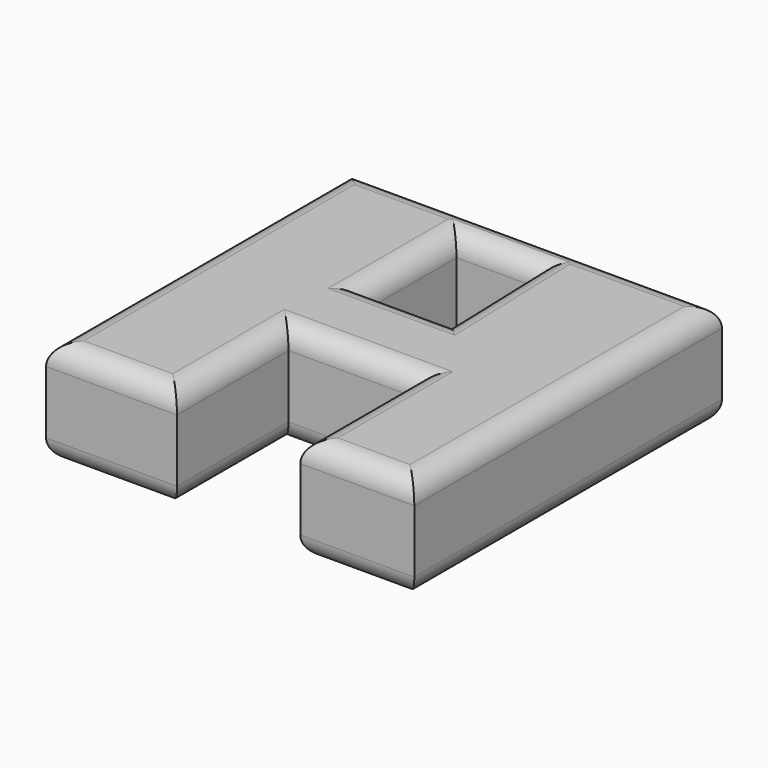
from build123d import *

# Parameters (mm, degrees)
F1_DEPTH      = 15
F2_T1_DEPTH   = 68.2414875925
F2_T3_DEPTH   = 69.4962510467
F2_T5_DEPTH   = 33.7555244192
F2_T7_DEPTH   = 27.4655555189
F2_T9_DEPTH   = 18.1505084038
F2_T11_DEPTH  = 28.0705761909
F2_T13_DEPTH  = 31.3354547694
F2_T15_DEPTH  = 70.1012717187
F2_T17_DEPTH  = 16.2727097049
F2_T22_DEPTH  = 19.0483759437
F2_T27_DEPTH  = 31.281174035
F2_T33_DEPTH  = 19.5733014774
F2_T38_DEPTH  = 19.0483759437
F2_T43_DEPTH  = 31.281174035
F2_T49_DEPTH  = 19.5733014774
F2_T55_DEPTH  = 25.6505084038
F2_T59_DEPTH  = 34.9655555189
F2_T66_DEPTH  = 35.5705761909
F2_T70_DEPTH  = 25.6505084038
F2_T77_DEPTH  = 23.7727097049
F2_T81_DEPTH  = 26.5483759437
F2_T88_DEPTH  = 31.281174035
F2_T92_DEPTH  = 19.0483759437
F2_T99_DEPTH  = 19.5733014774
F2_T103_DEPTH = 31.281174035
F2_T110_DEPTH = 23.7727097049
F2_T114_DEPTH = 27.0733014774
F2_T121_DEPTH = 34.9655555189
F2_T125_DEPTH = 25.6505084038
F2_T132_DEPTH = 25.6505084038
F2_T136_DEPTH = 35.5705761909
F2_T143_DEPTH = 26.5483759437
F2_T147_DEPTH = 23.7727097049
F2_T154_DEPTH = 19.0483759437
F2_T158_DEPTH = 31.281174035
F2_T165_DEPTH = 31.281174035
F2_T169_DEPTH = 19.5733014774
F2_T176_DEPTH = 27.0733014774
F2_T180_DEPTH = 23.7727097049


# Not quite as in the source:
# - a fillet or chamfer that OpenCascade refuses, or shapes differently, is made with other operations: its cross-section is extruded or revolved along the edge and cut away or added


with BuildPart() as f1:
    # F0 (on Top) → F1 (new body)
    with BuildSketch(Plane.XY):
        Polygon((24.4360174984, 0), (0, 0), (-25.7803853601, 0), (-28.8054700941, 0), (-28.8054700941, -54.4962510467), (-10.0499456748, -54.4962510467), (-10.0499456748, -34.5306955278), (8.1005627289, -34.5306955278), (8.1005627289, -55.1012717187), (24.4360174984, -55.1012717187), align=None)
        Polygon((-9.4178915024, -5.2225748077), (2.1304844413, -5.2225748077), (2.655409975, -21.4952845126), (-9.4178915024, -21.4952845126), align=None, mode=Mode.SUBTRACT)
    extrude(amount=F1_DEPTH)

    # F2: fillet of radius 3 on 24 edges, made by hand

    # F2_s2 → F2_t1 (cut)
    with BuildSketch(Plane.YZ.offset(-36.3054700941)):
        with BuildLine():
            ThreePointArc((0, 12), (-0.8786796564, 14.1213203436), (-3, 15))
            Line((-3, 15), (0, 15))
            Line((0, 15), (0, 12))
        make_face()
        with BuildLine():
            ThreePointArc((0, 3), (-0.8786796564, 0.8786796564), (-3, 0))
            Line((-3, 0), (0, 0))
            Line((0, 0), (0, 3))
        make_face()
    extrude(amount=F2_T1_DEPTH, mode=Mode.SUBTRACT)

    # F2_s4 → F2_t3 (cut)
    with BuildSketch(Plane.XZ.offset(-7.5)):
        with BuildLine():
            ThreePointArc((-28.8054700941, 12), (-27.9267904376, 14.1213203436), (-25.8054700941, 15))
            Line((-25.8054700941, 15), (-28.8054700941, 15))
            Line((-28.8054700941, 15), (-28.8054700941, 12))
        make_face()
        with BuildLine():
            ThreePointArc((-25.8054700941, 0), (-27.9267904376, 0.8786796564), (-28.8054700941, 3))
            Line((-28.8054700941, 3), (-28.8054700941, 0))
            Line((-28.8054700941, 0), (-25.8054700941, 0))
        make_face()
    extrude(amount=F2_T3_DEPTH, mode=Mode.SUBTRACT)

    # F2_s6 → F2_t5 (cut)
    with BuildSketch(Plane.YZ.offset(-36.3054700941)):
        with BuildLine():
            ThreePointArc((-54.4962510467, 12), (-53.6175713902, 14.1213203436), (-51.4962510467, 15))
            Line((-51.4962510467, 15), (-54.4962510467, 15))
            Line((-54.4962510467, 15), (-54.4962510467, 12))
        make_face()
        with BuildLine():
            ThreePointArc((-51.4962510467, 0), (-53.6175713902, 0.8786796564), (-54.4962510467, 3))
            Line((-54.4962510467, 3), (-54.4962510467, 0))
            Line((-54.4962510467, 0), (-51.4962510467, 0))
        make_face()
    extrude(amount=F2_T5_DEPTH, mode=Mode.SUBTRACT)

    # F2_s8 → F2_t7 (cut)
    with BuildSketch(Plane.XZ.offset(34.5306955278)):
        with BuildLine():
            ThreePointArc((-10.0499456748, 12), (-10.9286253313, 14.1213203436), (-13.0499456748, 15))
            Line((-13.0499456748, 15), (-10.0499456748, 15))
            Line((-10.0499456748, 15), (-10.0499456748, 12))
        make_face()
        with BuildLine():
            ThreePointArc((-13.0499456748, 0), (-10.9286253313, 0.8786796564), (-10.0499456748, 3))
            Line((-10.0499456748, 3), (-10.0499456748, 0))
            Line((-10.0499456748, 0), (-13.0499456748, 0))
        make_face()
    extrude(amount=F2_T7_DEPTH, mode=Mode.SUBTRACT)

    # F2_s10 → F2_t9 (cut)
    with BuildSketch(Plane.YZ.offset(-10.0499456748)):
        with BuildLine():
            ThreePointArc((-34.5306955278, 12), (-33.6520158714, 14.1213203436), (-31.5306955278, 15))
            Line((-31.5306955278, 15), (-34.5306955278, 15))
            Line((-34.5306955278, 15), (-34.5306955278, 12))
        make_face()
        with BuildLine():
            ThreePointArc((-31.5306955278, 0), (-33.6520158714, 0.8786796564), (-34.5306955278, 3))
            Line((-34.5306955278, 3), (-34.5306955278, 0))
            Line((-34.5306955278, 0), (-31.5306955278, 0))
        make_face()
    extrude(amount=F2_T9_DEPTH, mode=Mode.SUBTRACT)

    # F2_s12 → F2_t11 (cut)
    with BuildSketch(Plane.XZ.offset(34.5306955278)):
        with BuildLine():
            ThreePointArc((8.1005627289, 12), (8.9792423854, 14.1213203436), (11.1005627289, 15))
            Line((11.1005627289, 15), (8.1005627289, 15))
            Line((8.1005627289, 15), (8.1005627289, 12))
        make_face()
        with BuildLine():
            ThreePointArc((11.1005627289, 0), (8.9792423854, 0.8786796564), (8.1005627289, 3))
            Line((8.1005627289, 3), (8.1005627289, 0))
            Line((8.1005627289, 0), (11.1005627289, 0))
        make_face()
    extrude(amount=F2_T11_DEPTH, mode=Mode.SUBTRACT)

    # F2_s14 → F2_t13 (cut)
    with BuildSketch(Plane.YZ.offset(0.6005627289)):
        with BuildLine():
            ThreePointArc((-55.1012717187, 12), (-54.2225920623, 14.1213203436), (-52.1012717187, 15))
            Line((-52.1012717187, 15), (-55.1012717187, 15))
            Line((-55.1012717187, 15), (-55.1012717187, 12))
        make_face()
        with BuildLine():
            ThreePointArc((-52.1012717187, 0), (-54.2225920623, 0.8786796564), (-55.1012717187, 3))
            Line((-55.1012717187, 3), (-55.1012717187, 0))
            Line((-55.1012717187, 0), (-52.1012717187, 0))
        make_face()
    extrude(amount=F2_T13_DEPTH, mode=Mode.SUBTRACT)

    # F2_s16 → F2_t15 (cut)
    with BuildSketch(Plane.XZ.offset(-7.5)):
        with BuildLine():
            ThreePointArc((21.4360174984, 15), (23.5573378419, 14.1213203436), (24.4360174984, 12))
            Line((24.4360174984, 12), (24.4360174984, 15))
            Line((24.4360174984, 15), (21.4360174984, 15))
        make_face()
        with BuildLine():
            ThreePointArc((21.4360174984, 0), (23.5573378419, 0.8786796564), (24.4360174984, 3))
            Line((24.4360174984, 3), (24.4360174984, 0))
            Line((24.4360174984, 0), (21.4360174984, 0))
        make_face()
    extrude(amount=F2_T15_DEPTH, mode=Mode.SUBTRACT)

    # F2_s18 → F2_t17 (cut)
    with BuildSketch(Plane.XZ.offset(5.2225748077)):
        with BuildLine():
            ThreePointArc((-9.4178915024, 12), (-10.2965711588, 14.1213203436), (-12.4178915024, 15))
            Line((-12.4178915024, 15), (-9.4178915024, 15))
            Line((-9.4178915024, 15), (-9.4178915024, 12))
        make_face()
        with BuildLine():
            ThreePointArc((-12.4178915024, 0), (-10.2965711588, 0.8786796564), (-9.4178915024, 3))
            Line((-9.4178915024, 3), (-9.4178915024, 0))
            Line((-9.4178915024, 0), (-12.4178915024, 0))
        make_face()
    extrude(amount=F2_T17_DEPTH, mode=Mode.SUBTRACT)


with BuildPart() as f2_tool20:
    # F2_s21 → F2_t22 (new body)
    with BuildSketch(Plane.YZ.offset(-9.4178915024)):
        with BuildLine():
            ThreePointArc((-5.2225748077, 12), (-4.3438951513, 14.1213203436), (-2.2225748077, 15))
            Line((-2.2225748077, 15), (-5.2225748077, 15))
            Line((-5.2225748077, 15), (-5.2225748077, 12))
        make_face()
    extrude(amount=F2_T22_DEPTH)

    split(bisect_by=Plane(origin=(1.9599749627, 0.0632249282, 0), x_dir=(0, 0, 1), z_dir=(-0.9994801155, -0.0322412581, 0)), keep=Keep.TOP)


with BuildPart() as f1_1:
    add(f1.part)

    # F2_t19: cut F2_tool20
    add(f2_tool20.part, mode=Mode.SUBTRACT)


with BuildPart() as f2_tool25:
    # F2_s26 → F2_t27 (new body)
    with BuildSketch(Plane(origin=(-0.0712999569, 2.2103011303, 0), x_dir=(0, 0, 1), z_dir=(0.0322412581, -0.9994801155, 0))):
        with BuildLine():
            ThreePointArc((12, -1.9609944533), (14.1213203436, -2.8396741098), (15, -4.9609944533))
            Line((15, -4.9609944533), (15, -1.9609944533))
            Line((15, -1.9609944533), (12, -1.9609944533))
        make_face()
    extrude(amount=F2_T27_DEPTH)

    split(bisect_by=Plane.XZ.offset(21.4952845126), keep=Keep.BOTTOM)

    split(bisect_by=Plane.XZ.offset(5.2225748077), keep=Keep.TOP)


with BuildPart() as f1_2:
    add(f1_1.part)

    # F2_t24: cut F2_tool25
    add(f2_tool25.part, mode=Mode.SUBTRACT)


with BuildPart() as f2_tool31:
    # F2_s32 → F2_t33 (new body)
    with BuildSketch(Plane.YZ.offset(10.155409975)):
        with BuildLine():
            ThreePointArc((-21.4952845126, 12), (-22.3739641691, 14.1213203436), (-24.4952845126, 15))
            Line((-24.4952845126, 15), (-21.4952845126, 15))
            Line((-21.4952845126, 15), (-21.4952845126, 12))
        make_face()
    extrude(amount=-F2_T33_DEPTH)

    split(bisect_by=Plane(origin=(1.9599749627, 0.0632249282, 0), x_dir=(0, 0, 1), z_dir=(-0.9994801155, -0.0322412581, 0)), keep=Keep.TOP)


with BuildPart() as f1_3:
    add(f1_2.part)

    # F2_t30: cut F2_tool31
    add(f2_tool31.part, mode=Mode.SUBTRACT)


with BuildPart() as f2_tool36:
    # F2_s37 → F2_t38 (new body)
    with BuildSketch(Plane.YZ.offset(-9.4178915024)):
        with BuildLine():
            ThreePointArc((-2.2225748077, 0), (-4.3438951513, 0.8786796564), (-5.2225748077, 3))
            Line((-5.2225748077, 3), (-5.2225748077, 0))
            Line((-5.2225748077, 0), (-2.2225748077, 0))
        make_face()
    extrude(amount=F2_T38_DEPTH)

    split(bisect_by=Plane(origin=(1.9599749627, 0.0632249282, 0), x_dir=(0, 0, 1), z_dir=(-0.9994801155, -0.0322412581, 0)), keep=Keep.TOP)


with BuildPart() as f1_4:
    add(f1_3.part)

    # F2_t35: cut F2_tool36
    add(f2_tool36.part, mode=Mode.SUBTRACT)


with BuildPart() as f2_tool41:
    # F2_s42 → F2_t43 (new body)
    with BuildSketch(Plane(origin=(-0.0712999569, 2.2103011303, 0), x_dir=(0, 0, 1), z_dir=(0.0322412581, -0.9994801155, 0))):
        with BuildLine():
            ThreePointArc((0, -4.9609944533), (0.8786796564, -2.8396741098), (3, -1.9609944533))
            Line((3, -1.9609944533), (0, -1.9609944533))
            Line((0, -1.9609944533), (0, -4.9609944533))
        make_face()
    extrude(amount=F2_T43_DEPTH)

    split(bisect_by=Plane.XZ.offset(21.4952845126), keep=Keep.BOTTOM)

    split(bisect_by=Plane.XZ.offset(5.2225748077), keep=Keep.TOP)


with BuildPart() as f1_5:
    add(f1_4.part)

    # F2_t40: cut F2_tool41
    add(f2_tool41.part, mode=Mode.SUBTRACT)


with BuildPart() as f2_tool47:
    # F2_s48 → F2_t49 (new body)
    with BuildSketch(Plane.YZ.offset(10.155409975)):
        with BuildLine():
            ThreePointArc((-24.4952845126, 0), (-22.3739641691, 0.8786796564), (-21.4952845126, 3))
            Line((-21.4952845126, 3), (-21.4952845126, 0))
            Line((-21.4952845126, 0), (-24.4952845126, 0))
        make_face()
    extrude(amount=-F2_T49_DEPTH)

    split(bisect_by=Plane(origin=(1.9599749627, 0.0632249282, 0), x_dir=(0, 0, 1), z_dir=(-0.9994801155, -0.0322412581, 0)), keep=Keep.TOP)


with BuildPart() as f1_6:
    add(f1_5.part)

    # F2_t46: cut F2_tool47
    add(f2_tool47.part, mode=Mode.SUBTRACT)


with BuildPart() as f2_tool53:
    # F2_s54 → F2_t55 (new body)
    with BuildSketch(Plane.YZ.offset(-17.5499456748)):
        with BuildLine():
            ThreePointArc((-34.5306955278, 12), (-33.6520158714, 14.1213203436), (-31.5306955278, 15))
            Line((-31.5306955278, 15), (-34.5306955278, 15))
            Line((-34.5306955278, 15), (-34.5306955278, 12))
        make_face()
    extrude(amount=F2_T55_DEPTH)

    split(bisect_by=Plane.YZ.offset(-10.0499456748), keep=Keep.BOTTOM)


with BuildPart() as f2_tool57:
    # F2_s58 → F2_t59 (new body)
    with BuildSketch(Plane.XZ.offset(61.9962510467)):
        with BuildLine():
            ThreePointArc((-10.0499456748, 12), (-10.9286253313, 14.1213203436), (-13.0499456748, 15))
            Line((-13.0499456748, 15), (-10.0499456748, 15))
            Line((-10.0499456748, 15), (-10.0499456748, 12))
        make_face()
    extrude(amount=-F2_T59_DEPTH)

    split(bisect_by=Plane.XZ.offset(34.5306955278), keep=Keep.BOTTOM)


with BuildPart() as f2_tool53_1:
    add(f2_tool53.part)

    # F2_t61: intersect F2_tool57
    add(f2_tool57.part, mode=Mode.INTERSECT)


with BuildPart() as f1_7:
    add(f1_6.part)

    # F2_t51: cut F2_tool53
    add(f2_tool53_1.part, mode=Mode.SUBTRACT)


with BuildPart() as f2_tool64:
    # F2_s65 → F2_t66 (new body)
    with BuildSketch(Plane.XZ.offset(27.0306955278)):
        with BuildLine():
            ThreePointArc((8.1005627289, 12), (8.9792423854, 14.1213203436), (11.1005627289, 15))
            Line((11.1005627289, 15), (8.1005627289, 15))
            Line((8.1005627289, 15), (8.1005627289, 12))
        make_face()
    extrude(amount=F2_T66_DEPTH)

    split(bisect_by=Plane.XZ.offset(34.5306955278), keep=Keep.BOTTOM)


with BuildPart() as f2_tool68:
    # F2_s69 → F2_t70 (new body)
    with BuildSketch(Plane.YZ.offset(-10.0499456748)):
        with BuildLine():
            ThreePointArc((-34.5306955278, 12), (-33.6520158714, 14.1213203436), (-31.5306955278, 15))
            Line((-31.5306955278, 15), (-34.5306955278, 15))
            Line((-34.5306955278, 15), (-34.5306955278, 12))
        make_face()
    extrude(amount=F2_T70_DEPTH)

    split(bisect_by=Plane.YZ.offset(8.1005627289), keep=Keep.TOP)


with BuildPart() as f2_tool64_1:
    add(f2_tool64.part)

    # F2_t72: intersect F2_tool68
    add(f2_tool68.part, mode=Mode.INTERSECT)


with BuildPart() as f1_8:
    add(f1_7.part)

    # F2_t62: cut F2_tool64
    add(f2_tool64_1.part, mode=Mode.SUBTRACT)


with BuildPart() as f2_tool75:
    # F2_s76 → F2_t77 (new body)
    with BuildSketch(Plane.XZ.offset(21.4952845126)):
        with BuildLine():
            ThreePointArc((-9.4178915024, 12), (-10.2965711588, 14.1213203436), (-12.4178915024, 15))
            Line((-12.4178915024, 15), (-9.4178915024, 15))
            Line((-9.4178915024, 15), (-9.4178915024, 12))
        make_face()
    extrude(amount=-F2_T77_DEPTH)

    split(bisect_by=Plane.XZ.offset(5.2225748077), keep=Keep.BOTTOM)


with BuildPart() as f2_tool79:
    # F2_s80 → F2_t81 (new body)
    with BuildSketch(Plane.YZ.offset(-16.9178915024)):
        with BuildLine():
            ThreePointArc((-5.2225748077, 12), (-4.3438951513, 14.1213203436), (-2.2225748077, 15))
            Line((-2.2225748077, 15), (-5.2225748077, 15))
            Line((-5.2225748077, 15), (-5.2225748077, 12))
        make_face()
    extrude(amount=F2_T81_DEPTH)

    split(bisect_by=Plane.YZ.offset(-9.4178915024), keep=Keep.BOTTOM)


with BuildPart() as f2_tool75_1:
    add(f2_tool75.part)

    # F2_t83: intersect F2_tool79
    add(f2_tool79.part, mode=Mode.INTERSECT)


with BuildPart() as f1_9:
    add(f1_8.part)

    # F2_t73: cut F2_tool75
    add(f2_tool75_1.part, mode=Mode.SUBTRACT)


with BuildPart() as f2_tool86:
    # F2_s87 → F2_t88 (new body)
    with BuildSketch(Plane(origin=(-0.0712999569, 2.2103011303, 0), x_dir=(0, 0, 1), z_dir=(0.0322412581, -0.9994801155, 0))):
        with BuildLine():
            ThreePointArc((12, -1.9609944533), (14.1213203436, -2.8396741098), (15, -4.9609944533))
            Line((15, -4.9609944533), (15, -1.9609944533))
            Line((15, -1.9609944533), (12, -1.9609944533))
        make_face()
    extrude(amount=F2_T88_DEPTH)

    split(bisect_by=Plane.XZ.offset(5.2225748077), keep=Keep.BOTTOM)


with BuildPart() as f2_tool90:
    # F2_s91 → F2_t92 (new body)
    with BuildSketch(Plane.YZ.offset(-9.4178915024)):
        with BuildLine():
            ThreePointArc((-5.2225748077, 12), (-4.3438951513, 14.1213203436), (-2.2225748077, 15))
            Line((-2.2225748077, 15), (-5.2225748077, 15))
            Line((-5.2225748077, 15), (-5.2225748077, 12))
        make_face()
    extrude(amount=F2_T92_DEPTH)

    split(bisect_by=Plane(origin=(1.9599749627, 0.0632249282, 0), x_dir=(0, 0, 1), z_dir=(0.9994801155, 0.0322412581, 0)), keep=Keep.TOP)


with BuildPart() as f2_tool86_1:
    add(f2_tool86.part)

    # F2_t94: intersect F2_tool90
    add(f2_tool90.part, mode=Mode.INTERSECT)


with BuildPart() as f1_10:
    add(f1_9.part)

    # F2_t84: cut F2_tool86
    add(f2_tool86_1.part, mode=Mode.SUBTRACT)


with BuildPart() as f2_tool97:
    # F2_s98 → F2_t99 (new body)
    with BuildSketch(Plane.YZ.offset(10.155409975)):
        with BuildLine():
            ThreePointArc((-21.4952845126, 12), (-22.3739641691, 14.1213203436), (-24.4952845126, 15))
            Line((-24.4952845126, 15), (-21.4952845126, 15))
            Line((-21.4952845126, 15), (-21.4952845126, 12))
        make_face()
    extrude(amount=-F2_T99_DEPTH)

    split(bisect_by=Plane(origin=(1.9599749627, 0.0632249282, 0), x_dir=(0, 0, 1), z_dir=(0.9994801155, 0.0322412581, 0)), keep=Keep.TOP)


with BuildPart() as f2_tool101:
    # F2_s102 → F2_t103 (new body)
    with BuildSketch(Plane(origin=(-0.0712999569, 2.2103011303, 0), x_dir=(0, 0, 1), z_dir=(0.0322412581, -0.9994801155, 0))):
        with BuildLine():
            ThreePointArc((12, -1.9609944533), (14.1213203436, -2.8396741098), (15, -4.9609944533))
            Line((15, -4.9609944533), (15, -1.9609944533))
            Line((15, -1.9609944533), (12, -1.9609944533))
        make_face()
    extrude(amount=F2_T103_DEPTH)

    split(bisect_by=Plane.XZ.offset(21.4952845126), keep=Keep.TOP)


with BuildPart() as f2_tool97_1:
    add(f2_tool97.part)

    # F2_t105: intersect F2_tool101
    add(f2_tool101.part, mode=Mode.INTERSECT)


with BuildPart() as f1_11:
    add(f1_10.part)

    # F2_t95: cut F2_tool97
    add(f2_tool97_1.part, mode=Mode.SUBTRACT)


with BuildPart() as f2_tool108:
    # F2_s109 → F2_t110 (new body)
    with BuildSketch(Plane.XZ.offset(28.9952845126)):
        with BuildLine():
            ThreePointArc((-9.4178915024, 12), (-10.2965711588, 14.1213203436), (-12.4178915024, 15))
            Line((-12.4178915024, 15), (-9.4178915024, 15))
            Line((-9.4178915024, 15), (-9.4178915024, 12))
        make_face()
    extrude(amount=-F2_T110_DEPTH)

    split(bisect_by=Plane.XZ.offset(21.4952845126), keep=Keep.TOP)


with BuildPart() as f2_tool112:
    # F2_s113 → F2_t114 (new body)
    with BuildSketch(Plane.YZ.offset(10.155409975)):
        with BuildLine():
            ThreePointArc((-21.4952845126, 12), (-22.3739641691, 14.1213203436), (-24.4952845126, 15))
            Line((-24.4952845126, 15), (-21.4952845126, 15))
            Line((-21.4952845126, 15), (-21.4952845126, 12))
        make_face()
    extrude(amount=-F2_T114_DEPTH)

    split(bisect_by=Plane.YZ.offset(-9.4178915024), keep=Keep.BOTTOM)


with BuildPart() as f2_tool108_1:
    add(f2_tool108.part)

    # F2_t116: intersect F2_tool112
    add(f2_tool112.part, mode=Mode.INTERSECT)


with BuildPart() as f1_12:
    add(f1_11.part)

    # F2_t106: cut F2_tool108
    add(f2_tool108_1.part, mode=Mode.SUBTRACT)


with BuildPart() as f2_tool119:
    # F2_s120 → F2_t121 (new body)
    with BuildSketch(Plane.XZ.offset(61.9962510467)):
        with BuildLine():
            ThreePointArc((-13.0499456748, 0), (-10.9286253313, 0.8786796564), (-10.0499456748, 3))
            Line((-10.0499456748, 3), (-10.0499456748, 0))
            Line((-10.0499456748, 0), (-13.0499456748, 0))
        make_face()
    extrude(amount=-F2_T121_DEPTH)

    split(bisect_by=Plane.XZ.offset(34.5306955278), keep=Keep.BOTTOM)


with BuildPart() as f2_tool123:
    # F2_s124 → F2_t125 (new body)
    with BuildSketch(Plane.YZ.offset(-17.5499456748)):
        with BuildLine():
            ThreePointArc((-31.5306955278, 0), (-33.6520158714, 0.8786796564), (-34.5306955278, 3))
            Line((-34.5306955278, 3), (-34.5306955278, 0))
            Line((-34.5306955278, 0), (-31.5306955278, 0))
        make_face()
    extrude(amount=F2_T125_DEPTH)

    split(bisect_by=Plane.YZ.offset(-10.0499456748), keep=Keep.BOTTOM)


with BuildPart() as f2_tool119_1:
    add(f2_tool119.part)

    # F2_t127: intersect F2_tool123
    add(f2_tool123.part, mode=Mode.INTERSECT)


with BuildPart() as f1_13:
    add(f1_12.part)

    # F2_t117: cut F2_tool119
    add(f2_tool119_1.part, mode=Mode.SUBTRACT)


with BuildPart() as f2_tool130:
    # F2_s131 → F2_t132 (new body)
    with BuildSketch(Plane.YZ.offset(-10.0499456748)):
        with BuildLine():
            ThreePointArc((-31.5306955278, 0), (-33.6520158714, 0.8786796564), (-34.5306955278, 3))
            Line((-34.5306955278, 3), (-34.5306955278, 0))
            Line((-34.5306955278, 0), (-31.5306955278, 0))
        make_face()
    extrude(amount=F2_T132_DEPTH)

    split(bisect_by=Plane.YZ.offset(8.1005627289), keep=Keep.TOP)


with BuildPart() as f2_tool134:
    # F2_s135 → F2_t136 (new body)
    with BuildSketch(Plane.XZ.offset(27.0306955278)):
        with BuildLine():
            ThreePointArc((11.1005627289, 0), (8.9792423854, 0.8786796564), (8.1005627289, 3))
            Line((8.1005627289, 3), (8.1005627289, 0))
            Line((8.1005627289, 0), (11.1005627289, 0))
        make_face()
    extrude(amount=F2_T136_DEPTH)

    split(bisect_by=Plane.XZ.offset(34.5306955278), keep=Keep.BOTTOM)


with BuildPart() as f2_tool130_1:
    add(f2_tool130.part)

    # F2_t138: intersect F2_tool134
    add(f2_tool134.part, mode=Mode.INTERSECT)


with BuildPart() as f1_14:
    add(f1_13.part)

    # F2_t128: cut F2_tool130
    add(f2_tool130_1.part, mode=Mode.SUBTRACT)


with BuildPart() as f2_tool141:
    # F2_s142 → F2_t143 (new body)
    with BuildSketch(Plane.YZ.offset(-16.9178915024)):
        with BuildLine():
            ThreePointArc((-2.2225748077, 0), (-4.3438951513, 0.8786796564), (-5.2225748077, 3))
            Line((-5.2225748077, 3), (-5.2225748077, 0))
            Line((-5.2225748077, 0), (-2.2225748077, 0))
        make_face()
    extrude(amount=F2_T143_DEPTH)

    split(bisect_by=Plane.YZ.offset(-9.4178915024), keep=Keep.BOTTOM)


with BuildPart() as f2_tool145:
    # F2_s146 → F2_t147 (new body)
    with BuildSketch(Plane.XZ.offset(21.4952845126)):
        with BuildLine():
            ThreePointArc((-12.4178915024, 0), (-10.2965711588, 0.8786796564), (-9.4178915024, 3))
            Line((-9.4178915024, 3), (-9.4178915024, 0))
            Line((-9.4178915024, 0), (-12.4178915024, 0))
        make_face()
    extrude(amount=-F2_T147_DEPTH)

    split(bisect_by=Plane.XZ.offset(5.2225748077), keep=Keep.BOTTOM)


with BuildPart() as f2_tool141_1:
    add(f2_tool141.part)

    # F2_t149: intersect F2_tool145
    add(f2_tool145.part, mode=Mode.INTERSECT)


with BuildPart() as f1_15:
    add(f1_14.part)

    # F2_t139: cut F2_tool141
    add(f2_tool141_1.part, mode=Mode.SUBTRACT)


with BuildPart() as f2_tool152:
    # F2_s153 → F2_t154 (new body)
    with BuildSketch(Plane.YZ.offset(-9.4178915024)):
        with BuildLine():
            ThreePointArc((-2.2225748077, 0), (-4.3438951513, 0.8786796564), (-5.2225748077, 3))
            Line((-5.2225748077, 3), (-5.2225748077, 0))
            Line((-5.2225748077, 0), (-2.2225748077, 0))
        make_face()
    extrude(amount=F2_T154_DEPTH)

    split(bisect_by=Plane(origin=(1.9599749627, 0.0632249282, 0), x_dir=(0, 0, 1), z_dir=(0.9994801155, 0.0322412581, 0)), keep=Keep.TOP)


with BuildPart() as f2_tool156:
    # F2_s157 → F2_t158 (new body)
    with BuildSketch(Plane(origin=(-0.0712999569, 2.2103011303, 0), x_dir=(0, 0, 1), z_dir=(0.0322412581, -0.9994801155, 0))):
        with BuildLine():
            ThreePointArc((0, -4.9609944533), (0.8786796564, -2.8396741098), (3, -1.9609944533))
            Line((3, -1.9609944533), (0, -1.9609944533))
            Line((0, -1.9609944533), (0, -4.9609944533))
        make_face()
    extrude(amount=F2_T158_DEPTH)

    split(bisect_by=Plane.XZ.offset(5.2225748077), keep=Keep.BOTTOM)


with BuildPart() as f2_tool152_1:
    add(f2_tool152.part)

    # F2_t160: intersect F2_tool156
    add(f2_tool156.part, mode=Mode.INTERSECT)


with BuildPart() as f1_16:
    add(f1_15.part)

    # F2_t150: cut F2_tool152
    add(f2_tool152_1.part, mode=Mode.SUBTRACT)


with BuildPart() as f2_tool163:
    # F2_s164 → F2_t165 (new body)
    with BuildSketch(Plane(origin=(-0.0712999569, 2.2103011303, 0), x_dir=(0, 0, 1), z_dir=(0.0322412581, -0.9994801155, 0))):
        with BuildLine():
            ThreePointArc((0, -4.9609944533), (0.8786796564, -2.8396741098), (3, -1.9609944533))
            Line((3, -1.9609944533), (0, -1.9609944533))
            Line((0, -1.9609944533), (0, -4.9609944533))
        make_face()
    extrude(amount=F2_T165_DEPTH)

    split(bisect_by=Plane.XZ.offset(21.4952845126), keep=Keep.TOP)


with BuildPart() as f2_tool167:
    # F2_s168 → F2_t169 (new body)
    with BuildSketch(Plane.YZ.offset(10.155409975)):
        with BuildLine():
            ThreePointArc((-24.4952845126, 0), (-22.3739641691, 0.8786796564), (-21.4952845126, 3))
            Line((-21.4952845126, 3), (-21.4952845126, 0))
            Line((-21.4952845126, 0), (-24.4952845126, 0))
        make_face()
    extrude(amount=-F2_T169_DEPTH)

    split(bisect_by=Plane(origin=(1.9599749627, 0.0632249282, 0), x_dir=(0, 0, 1), z_dir=(0.9994801155, 0.0322412581, 0)), keep=Keep.TOP)


with BuildPart() as f2_tool163_1:
    add(f2_tool163.part)

    # F2_t171: intersect F2_tool167
    add(f2_tool167.part, mode=Mode.INTERSECT)


with BuildPart() as f1_17:
    add(f1_16.part)

    # F2_t161: cut F2_tool163
    add(f2_tool163_1.part, mode=Mode.SUBTRACT)


with BuildPart() as f2_tool174:
    # F2_s175 → F2_t176 (new body)
    with BuildSketch(Plane.YZ.offset(10.155409975)):
        with BuildLine():
            ThreePointArc((-24.4952845126, 0), (-22.3739641691, 0.8786796564), (-21.4952845126, 3))
            Line((-21.4952845126, 3), (-21.4952845126, 0))
            Line((-21.4952845126, 0), (-24.4952845126, 0))
        make_face()
    extrude(amount=-F2_T176_DEPTH)

    split(bisect_by=Plane.YZ.offset(-9.4178915024), keep=Keep.BOTTOM)


with BuildPart() as f2_tool178:
    # F2_s179 → F2_t180 (new body)
    with BuildSketch(Plane.XZ.offset(28.9952845126)):
        with BuildLine():
            ThreePointArc((-12.4178915024, 0), (-10.2965711588, 0.8786796564), (-9.4178915024, 3))
            Line((-9.4178915024, 3), (-9.4178915024, 0))
            Line((-9.4178915024, 0), (-12.4178915024, 0))
        make_face()
    extrude(amount=-F2_T180_DEPTH)

    split(bisect_by=Plane.XZ.offset(21.4952845126), keep=Keep.TOP)


with BuildPart() as f2_tool174_1:
    add(f2_tool174.part)

    # F2_t182: intersect F2_tool178
    add(f2_tool178.part, mode=Mode.INTERSECT)


with BuildPart() as f1_18:
    add(f1_17.part)

    # F2_t172: cut F2_tool174
    add(f2_tool174_1.part, mode=Mode.SUBTRACT)


solid = f1_18.part
